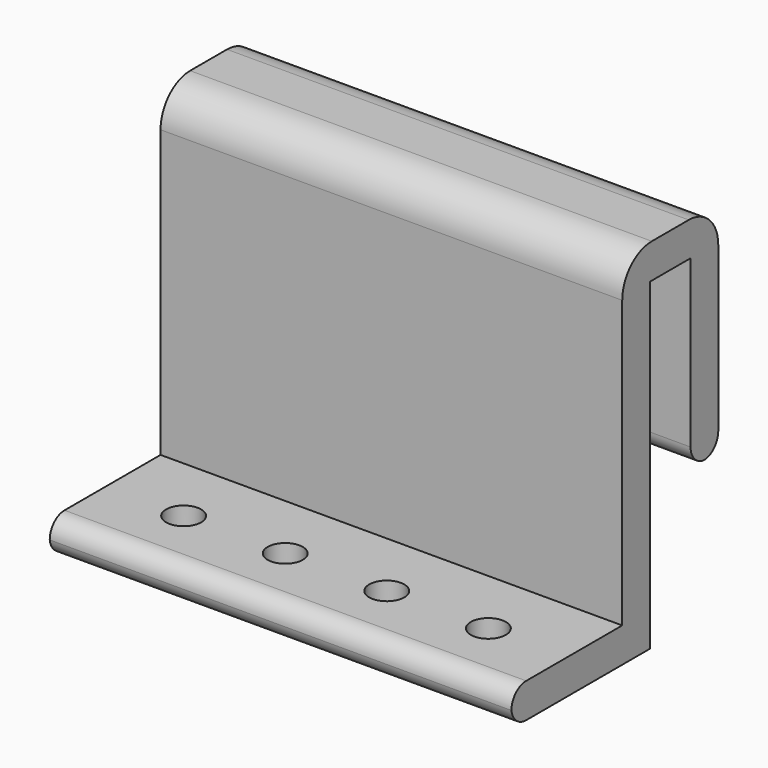
from build123d import *

# Parameters (mm, degrees)
F0_W         = 63.5
F0_H         = 25.4
F1_DEPTH     = 4.7625
F2_W         = 63.5
F2_H         = 16.51
F3_DEPTH     = 4.7625
F4_W         = 4.7625
F4_H         = 44.45
F5_DEPTH     = 63.5
F6_W         = 19.05
F6_H         = 4.7625
F7_DEPTH     = 63.5
F8_R         = 2.413
F9_DEPTH     = 4.7625
F10_R        = 5.08
F11_R        = 2.54
F12_T1_DEPTH = 76.2
F13_T1_DEPTH = 76.1003906189


# Not quite as in the source:
# - a fillet or chamfer that OpenCascade refuses, or shapes differently, is made with other operations: its cross-section is extruded or revolved along the edge and cut away or added


with BuildPart() as f1:
    # F0 (on Front) → F1 (new body)
    with BuildSketch(Plane.XZ):
        with Locations((-31.75, -12.7)):
            Rectangle(F0_W, F0_H)
    extrude(amount=F1_DEPTH)

    # F2 (on Top) → F3 (join)
    with BuildSketch(Plane.XY):
        with Locations((-31.75, -8.255)):
            Rectangle(F2_W, F2_H)
    extrude(amount=F3_DEPTH)

    # F4 (on Right) → F5 (join)
    with BuildSketch(Plane.YZ):
        with Locations((-14.12875, -22.225)):
            Rectangle(F4_W, F4_H)
    extrude(amount=-F5_DEPTH)

    # F6 (on Right) → F7 (join)
    with BuildSketch(Plane.YZ):
        with Locations((-26.035, -42.06875)):
            Rectangle(F6_W, F6_H)
    extrude(amount=-F7_DEPTH)

    # F8 (on face) → F9 (cut)
    with BuildSketch(Plane(origin=(0, 0, -44.45), x_dir=(1, 0, 0), z_dir=(0, 0, -1))):
        with Locations((-52.705, 26.035)):
            Circle(F8_R)
        with Locations((-38.735, 26.035)):
            Circle(F8_R)
        with Locations((-24.765, 26.035)):
            Circle(F8_R)
        with Locations((-10.795, 26.035)):
            Circle(F8_R)
    extrude(amount=-F9_DEPTH, mode=Mode.SUBTRACT)

    # F10
    f10_edges = [f1.edges().sort_by_distance(p)[0] for p in [
        (-31.75, 0, 4.7625),
        (-31.75, -16.51, 4.7625),
    ]]
    fillet(f10_edges, radius=F10_R)

    # F11
    f11_edges = [f1.edges().sort_by_distance(p)[0] for p in [
        (-31.75, -35.56, -39.6875),
    ]]
    fillet(f11_edges, radius=F11_R)

    # F12: fillet of radius 2.54 on 2 edges, made by hand

    # F12_s2 → F12_t1 (cut)
    with BuildSketch(Plane.YZ.offset(-69.85)):
        with BuildLine():
            ThreePointArc((-4.7625, -22.86), (-4.0185512242, -24.6560512242), (-2.2225, -25.4))
            Line((-2.2225, -25.4), (-4.7625, -25.4))
            Line((-4.7625, -25.4), (-4.7625, -22.86))
        make_face()
        with BuildLine():
            ThreePointArc((0, -22.86), (-0.7439487758, -24.6560512242), (-2.54, -25.4))
            Line((-2.54, -25.4), (0, -25.4))
            Line((0, -25.4), (0, -22.86))
        make_face()
    extrude(amount=F12_T1_DEPTH, mode=Mode.SUBTRACT)

    # F13: fillet of radius 2.54 on 1 edges, made by hand

    # F13_s2 → F13_t1 (cut)
    with BuildSketch(Plane.YZ.offset(-69.8001953095)):
        with BuildLine():
            ThreePointArc((-33.0399218762, -44.45), (-34.7199739587, -43.815), (-35.56, -42.2275))
            Line((-35.56, -42.2275), (-35.56, -44.45))
            Line((-35.56, -44.45), (-33.0399218762, -44.45))
        make_face()
    extrude(amount=F13_T1_DEPTH, mode=Mode.SUBTRACT)


solid = f1.part
